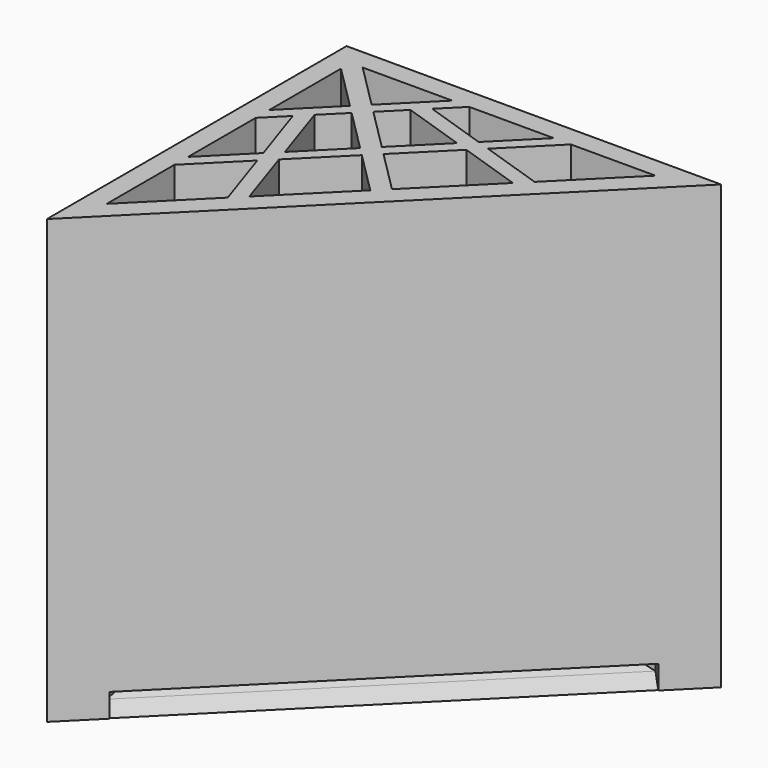
from build123d import *

# Parameters (mm, degrees)
F1_DEPTH    = 25
F2_SIZE2    = 24.99999
F2_SIZE     = 77.78174
F4_DEPTH    = 130
F5_W        = 126.5929291126
F5_H        = 5
F6_DEPTH    = 25
F7_T1_DEPTH = 126.5929291126
F9_DEPTH    = 15


# Not quite as in the source:
# - a fillet or chamfer that OpenCascade refuses, or shapes differently, is made with other operations: its cross-section is extruded or revolved along the edge and cut away or added
# - a fillet or chamfer is up to 0.001 mm smaller than in the source, because OpenCascade refuses the exact size


with BuildPart() as f1:
    # F0 (on Top) → F1 (new body)
    with BuildSketch(Plane.XY):
        Polygon((55, 55), (-55, 55), (-55, -55), align=None)
    extrude(amount=F1_DEPTH)

    # F2 (size 77.78175 and 25 in the source; OpenCascade refuses exactly that, so slightly less here)
    f2_edges = [f1.edges().sort_by_distance(p)[0] for p in [
        (0, 0, 25),
    ]]
    f2_side = f1.faces().sort_by_distance((-18.333333, 18.333333, 25))[0]
    chamfer(f2_edges, length=F2_SIZE, length2=F2_SIZE2, reference=f2_side)

    # F3 (on Top) → F4 (join)
    with BuildSketch(Plane.XY):
        Polygon((-55, 55), (-55, -55), (55, 55), align=None)
        Polygon((-49, -40.5147186258), (-49, 49), (40.5147186258, 49), align=None, mode=Mode.SUBTRACT)
    extrude(amount=F4_DEPTH)

    # F5 (on face) → F6 (cut)
    with BuildSketch(Plane(origin=(-4.2426406871, 4.2426406871, 0), x_dir=(-0.7071067812, -0.7071067812, 0), z_dir=(-0.7071067812, 0.7071067812, 0))):
        with Locations((0, 4.4284729387)):
            Rectangle(F5_W, F5_H)
    extrude(amount=-F6_DEPTH, mode=Mode.SUBTRACT)

    # F7: chamfer of 6 x 2 on 1 edges, made by hand

    # F7_s2 → F7_t1 (cut)
    with BuildSketch(Plane(origin=(44.7573593129, 44.7573593129, 0), x_dir=(0, 0, 1), z_dir=(-0.7071067812, -0.7071067812, 0))):
        Polygon((-0.0715270613, 0), (1.9284729387, 6), (1.9284729387, 0), align=None)
    extrude(amount=F7_T1_DEPTH, mode=Mode.SUBTRACT)

    # F8 (on face) → F9 (join)
    with BuildSketch(Plane.XY.offset(130)):
        Polygon((-45.4644660941, 49), (-49, 49), (-49, 45.4644660941), (-35.8485209767, 32.3129870708), (-49, 19.1615080475), (-49, 14.1615080475), (-42.9420274413, 20.2194806062), (-36.7324044532, 1.5906116418), (-49, -10.676983905), (-49, -15.676983905), (-35.4824044532, -2.1593883582), (-29.272970773, -20.7876893988), (-25.7374368671, -17.2521554928), (-31.9468705473, 1.3761455477), (-18.4292750005, 14.8937410945), (-6.0104076401, 2.4748737342), (-4.2426406871, 4.2426406871), (-2.4748737342, 6.0104076401), (-14.8937410945, 18.4292750005), (-1.3761455477, 31.9468705473), (17.2521554928, 25.7374368671), (20.7876893988, 29.272970773), (2.1593883582, 35.4824044532), (15.676983905, 49), (10.676983905, 49), (-1.5906116418, 36.7324044532), (-20.2194806062, 42.9420274413), (-14.1615080475, 49), (-19.1615080475, 49), (-32.3129870708, 35.8485209767), align=None)
        Polygon((-33.3485209767, 29.8129870708), (-20.9292750005, 17.3937410945), (-33.1968705473, 5.1261455477), (-39.4064935354, 23.7550145121), align=None, mode=Mode.SUBTRACT)
        Polygon((-17.3937410945, 20.9292750005), (-29.8129870708, 33.3485209767), (-23.7550145121, 39.4064935354), (-5.1261455477, 33.1968705473), align=None, mode=Mode.SUBTRACT)
    extrude(amount=-F9_DEPTH)


solid = f1.part
